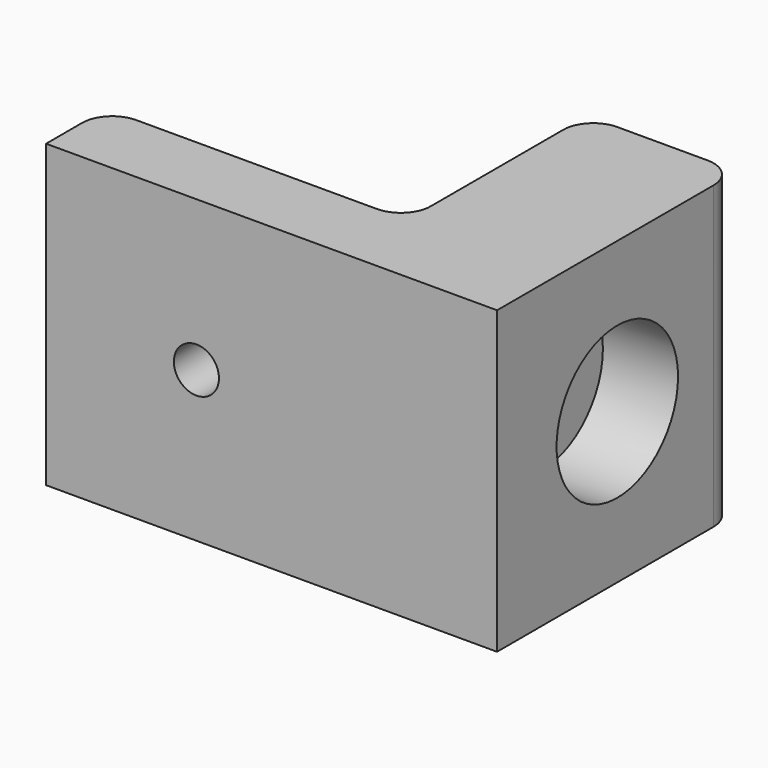
from build123d import *

# Parameters (mm, degrees)
F1_DEPTH     = 20
F2_R         = 5.05
F3_DEPTH     = 5
F4_R         = 1.5
F5_DEPTH     = 25
F6_R         = 2
F7_TEXT_SIZE = 4.2588587589
F8_DEPTH     = 0.4


# Not quite as in the source:
# - Text() gives the source's letters only with a copy of the font that has no kerning and outlines rounded to 1/6400 em; it was checked with that copy


with BuildPart() as f1:
    # F0 (on Top) → F1 (new body)
    with BuildSketch(Plane.XY):
        Polygon((20, 15), (20, 0), (0, 0), (0, -5), (30, -5), (30, 15), align=None)
    extrude(amount=F1_DEPTH)

    # F2 (on face) → F3 (cut)
    with BuildSketch(Plane.YZ.offset(30)):
        with Locations((5, 10)):
            Circle(F2_R)
    extrude(amount=-F3_DEPTH, mode=Mode.SUBTRACT)

    # F4 (on face) → F5 (cut)
    with BuildSketch(Plane(origin=(0, 0, 0), x_dir=(-1, 0, 0), z_dir=(0, 1, 0))):
        with Locations((-10, 10)):
            Circle(F4_R)
    extrude(amount=-F5_DEPTH, mode=Mode.SUBTRACT)

    # F6
    f6_edges = [f1.edges().sort_by_distance(p)[0] for p in [
        (20, 0, 10),
        (0, 0, 10),
        (30, 15, 10),
        (20, 15, 10),
    ]]
    fillet(f6_edges, radius=F6_R)


with BuildPart() as f8:
    # F7 (on face) → F8 (new body)
    with BuildSketch(Plane(origin=(0, 15, 0), x_dir=(-1, 0, 0), z_dir=(0, 1, 0))):
        with Locations(Location((-23.5, 2), (0, 0, 90))):
            Text('SIKORA', F7_TEXT_SIZE, font='Open Sans', font_style=FontStyle.BOLD, text_align=(TextAlign.LEFT, TextAlign.BOTTOM))
    extrude(amount=F8_DEPTH)


solid = Compound([f1.part, f8.part])
